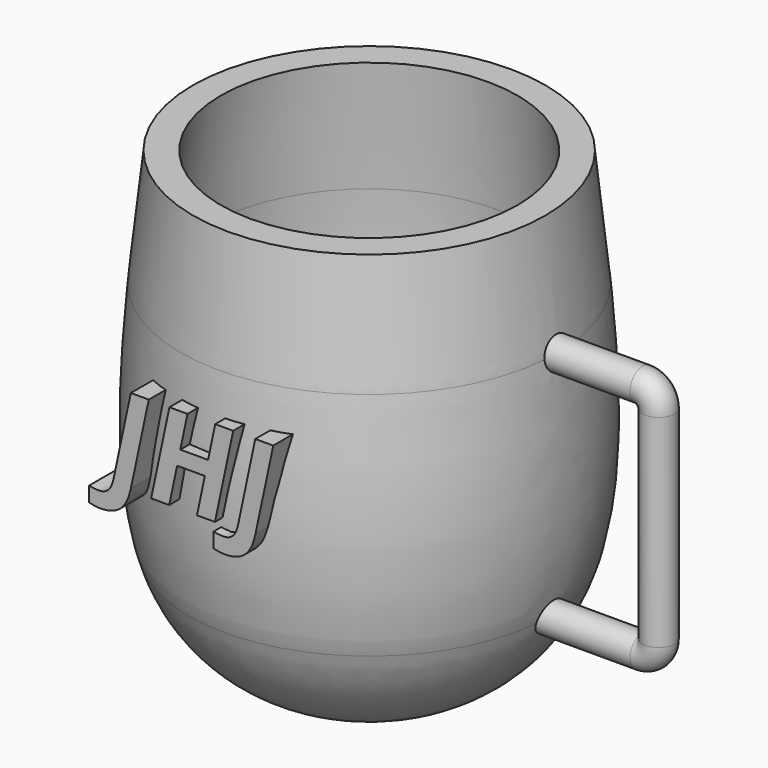
from build123d import *

# Parameters (mm, degrees)
F3_R         = 3.9548802034
F6_TEXT_SIZE = 30.2042618083
F7_DEPTH     = 10


# Not quite as in the source:
# - a feature names something its author has since deleted; it is built from what else it names
# - Text() gives the source's letters only with a copy of the font that has no kerning and outlines rounded to 1/6400 em; it was checked with that copy


with BuildPart() as f1:
    # F0 (on Front) → F1 (revolve)
    with BuildSketch(Plane.XZ):
        with BuildLine():
            add(Edge.make_bspline(
                [(39.8998260498, 16.9851593673), (39.1759500717, 26.7016865536), (38.1180710615, 36.6319908073), (37.1345591472, 46.2226457894)],
                knots=[0.6323891405, 0.6323891405, 0.6323891405, 0.6323891405, 0.758602804, 0.758602804, 0.758602804, 0.758602804], degree=3))
            Line((39.8998260498, 16.9851593673), (47.188355924, 16.9851593673))
            add(Edge.make_bspline(
                [(47.188355924, 16.9851593673), (46.2727992917, 26.754058711), (45.1157915675, 36.6508377878), (44.1208354225, 46.2226457894)],
                knots=[0.6610994407, 0.6610994407, 0.6610994407, 0.6610994407, 0.7779233136, 0.7779233136, 0.7779233136, 0.7779233136], degree=3))
            Line((44.1208354225, 46.2226457894), (37.1345591472, 46.2226457894))
        make_face()
        with BuildLine():
            add(Edge.make_bspline(
                [(0, -61.7330407779), (11.995163964, -61.875772615), (41.5520478298, -49.6769918097), (41.4051021183, -3.2200363917), (39.8998260498, 16.9851593673)],
                knots=[0, 0, 0, 0, 0.3699320165, 0.6323891405, 0.6323891405, 0.6323891405, 0.6323891405], degree=3))
            Line((0, -61.7330407779), (0, -70.7374885678))
            add(Edge.make_bspline(
                [(0, -70.7374885678), (13.6378493112, -74.3114916707), (36.3494046336, -65.9748152293), (44.6858964631, -43.1747716775), (45.1512640435, -41.7101274729)],
                knots=[0, 0, 0, 0, 0.374321855, 0.3990593816, 0.3990593816, 0.3990593816, 0.3990593816], degree=3))
            add(Edge.make_bspline(
                [(45.1512640435, -41.7101274729), (50.0808170295, -26.1954214279), (49.2419816779, -4.9268257286), (47.188355924, 16.9851593673)],
                knots=[0.3990593816, 0.3990593816, 0.3990593816, 0.3990593816, 0.6610994407, 0.6610994407, 0.6610994407, 0.6610994407], degree=3))
            Line((47.188355924, 16.9851593673), (39.8998260498, 16.9851593673))
        make_face()
    revolve(axis=Axis((0, 0, -7.014926523), (0, 0, 1)))

    # F4: sweep along a path in F0
    with BuildLine(Plane.XZ) as f4_path:
        Line((36.4107228816, -41.7101274729), (68.4248384833, -41.7101274729))
        ThreePointArc((68.4248384833, -41.7101274729), (71.2532656081, -40.5385545976), (72.4248384833, -37.7101274729))
        Line((72.4248384833, -37.7101274729), (72.4248384833, 12.9851593673))
        ThreePointArc((72.4248384833, 12.9851593673), (71.2532656081, 15.8135864921), (68.4248384833, 16.9851593673))
        Line((68.4248384833, 16.9851593673), (39.8998260498, 16.9851593673))
    # F3 (on line) → F4 (sweep)
    with BuildSketch(Plane.YZ.offset(39.8998260498)):
        with Locations((0, -41.7101274729)):
            Circle(F3_R)
    sweep(path=f4_path.line)


with BuildPart() as f7:
    # F6 (on offset) → F7 (new body)
    with BuildSketch(Plane.XZ.offset(41)):
        with Locations((-24.53456074, -14.1934342682)):
            Text('JHJ', F6_TEXT_SIZE, font='Open Sans', font_style=FontStyle.BOLDITALIC, text_align=(TextAlign.LEFT, TextAlign.BOTTOM))
    extrude(amount=F7_DEPTH)


solid = Compound([f1.part, f7.part])
